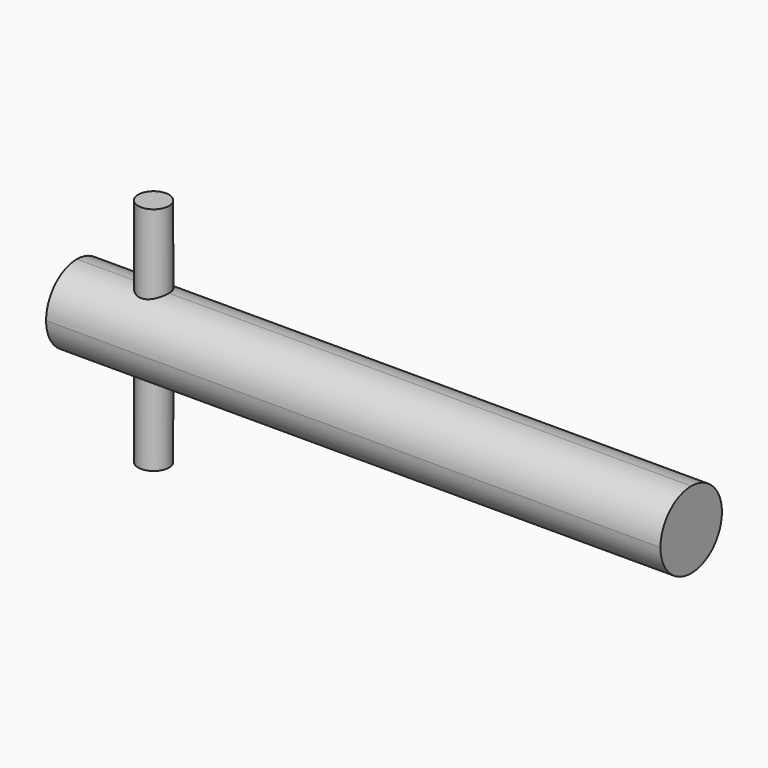
from build123d import *

# Parameters (mm, degrees)
F0_W         = 12.7
F0_H         = 12.7
F1_DEPTH     = 101.6
F2_R         = 2.54
F3_DEPTH     = 25.4
F4_DEPTH     = 12.7
F5_T4_DEPTH  = 133.35
F5_S5_R      = 2.54
F5_T6_DEPTH  = 68
F5_T10_DEPTH = 133.35
F5_S11_R     = 2.54
F5_T12_DEPTH = 68
F5_T16_DEPTH = 133.35
F5_S17_R     = 2.54
F5_T18_DEPTH = 68
F5_T22_DEPTH = 133.35
F5_S23_R     = 2.54
F5_T24_DEPTH = 68


# Not quite as in the source:
# - a fillet or chamfer that OpenCascade refuses, or shapes differently, is made with other operations: its cross-section is extruded or revolved along the edge and cut away or added


with BuildPart() as f1:
    # F0 (on Right) → F1 (new body)
    with BuildSketch(Plane.YZ):
        with Locations((-1.0797850298, 14.7537575103)):
            Rectangle(F0_W, F0_H)
    extrude(amount=F1_DEPTH)

    # F2 (on face) → F3 (join)
    with BuildSketch(Plane.XY.offset(21.1037575103)):
        with Locations((12.7, -1.0797850298)):
            Circle(F2_R)
    extrude(amount=-F3_DEPTH)

    # F2 (on face) → F4 (join)
    with BuildSketch(Plane.XY.offset(21.1037575103)):
        with Locations((12.7, -1.0797850298)):
            Circle(F2_R)
    extrude(amount=F4_DEPTH)

    # F5: fillet of radius 6.35 on 4 edges, made by hand


with BuildPart() as f5_tool2:
    # F5_s3 → F5_t4 (new body)
    with BuildSketch(Plane.YZ.offset(-15.875)):
        with BuildLine():
            ThreePointArc((-7.4297850298, 14.7537575103), (-5.5699130903, 19.2438855709), (-1.0797850298, 21.1037575103))
            Line((-1.0797850298, 21.1037575103), (-7.4297850298, 21.1037575103))
            Line((-7.4297850298, 21.1037575103), (-7.4297850298, 14.7537575103))
        make_face()
    extrude(amount=F5_T4_DEPTH)

    # F5_s5 → F5_t6 (cut, symmetric)
    with BuildSketch(Plane.XY.offset(17.9)):
        with Locations((12.7, -1.0797850298)):
            Circle(F5_S5_R)
    extrude(amount=F5_T6_DEPTH, both=True, mode=Mode.SUBTRACT)


with BuildPart() as f1_1:
    add(f1.part)

    # F5_t1: cut F5_tool2
    add(f5_tool2.part, mode=Mode.SUBTRACT)


with BuildPart() as f5_tool8:
    # F5_s9 → F5_t10 (new body)
    with BuildSketch(Plane.YZ.offset(-15.875)):
        with BuildLine():
            ThreePointArc((-1.0797850298, 21.1037575103), (3.4103430308, 19.2438855709), (5.2702149702, 14.7537575103))
            Line((5.2702149702, 14.7537575103), (5.2702149702, 21.1037575103))
            Line((5.2702149702, 21.1037575103), (-1.0797850298, 21.1037575103))
        make_face()
    extrude(amount=F5_T10_DEPTH)

    # F5_s11 → F5_t12 (cut, symmetric)
    with BuildSketch(Plane.XY.offset(17.9)):
        with Locations((12.7, -1.0797850298)):
            Circle(F5_S11_R)
    extrude(amount=F5_T12_DEPTH, both=True, mode=Mode.SUBTRACT)


with BuildPart() as f1_2:
    add(f1_1.part)

    # F5_t7: cut F5_tool8
    add(f5_tool8.part, mode=Mode.SUBTRACT)


with BuildPart() as f5_tool14:
    # F5_s15 → F5_t16 (new body)
    with BuildSketch(Plane.YZ.offset(-15.875)):
        with BuildLine():
            ThreePointArc((-7.4297850298, 14.7537575103), (-5.5699130903, 10.2636294498), (-1.0797850298, 8.4037575103))
            Line((-1.0797850298, 8.4037575103), (-7.4297850298, 8.4037575103))
            Line((-7.4297850298, 8.4037575103), (-7.4297850298, 14.7537575103))
        make_face()
    extrude(amount=F5_T16_DEPTH)

    # F5_s17 → F5_t18 (cut, symmetric)
    with BuildSketch(Plane.XY.offset(11.6)):
        with Locations((12.7, -1.0797850298)):
            Circle(F5_S17_R)
    extrude(amount=F5_T18_DEPTH, both=True, mode=Mode.SUBTRACT)


with BuildPart() as f1_3:
    add(f1_2.part)

    # F5_t13: cut F5_tool14
    add(f5_tool14.part, mode=Mode.SUBTRACT)


with BuildPart() as f5_tool20:
    # F5_s21 → F5_t22 (new body)
    with BuildSketch(Plane.YZ.offset(-15.875)):
        with BuildLine():
            ThreePointArc((-1.0797850298, 8.4037575103), (3.4103430308, 10.2636294498), (5.2702149702, 14.7537575103))
            Line((5.2702149702, 14.7537575103), (5.2702149702, 8.4037575103))
            Line((5.2702149702, 8.4037575103), (-1.0797850298, 8.4037575103))
        make_face()
    extrude(amount=F5_T22_DEPTH)

    # F5_s23 → F5_t24 (cut, symmetric)
    with BuildSketch(Plane.XY.offset(11.6)):
        with Locations((12.7, -1.0797850298)):
            Circle(F5_S23_R)
    extrude(amount=F5_T24_DEPTH, both=True, mode=Mode.SUBTRACT)


with BuildPart() as f1_4:
    add(f1_3.part)

    # F5_t19: cut F5_tool20
    add(f5_tool20.part, mode=Mode.SUBTRACT)


solid = f1_4.part
